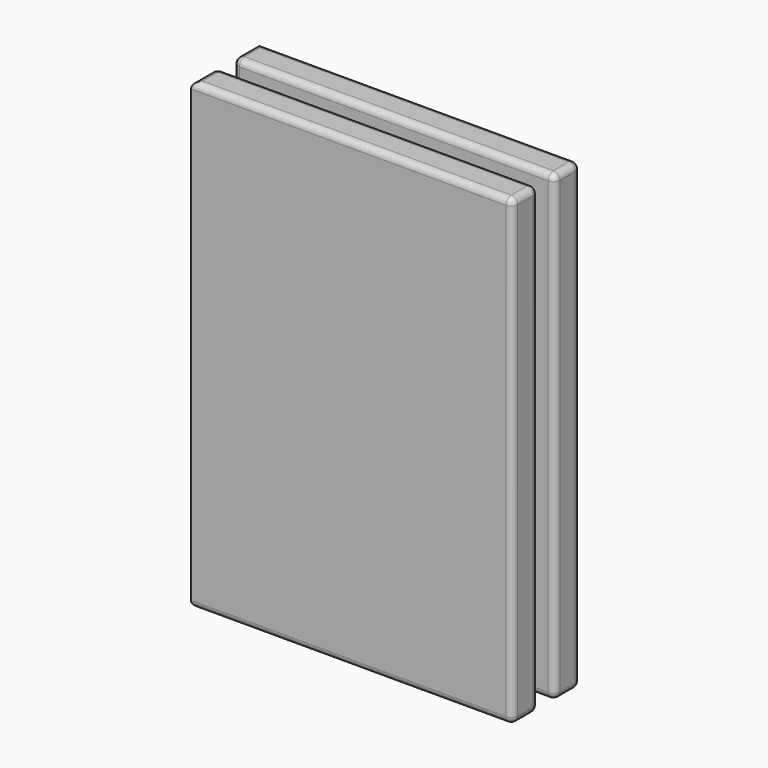
from build123d import *

# Parameters (mm, degrees)
F3_R     = 12.5
F4_DEPTH = 10
F6_DEPTH = 30
F7_R     = 5


with BuildPart() as f2:
    # F2: sweep along a path in F1
    with BuildLine(Plane.XZ) as f2_path:
        Line((0, 0), (250, 0))
    # F0 (on Right) → F2 (sweep)
    with BuildSketch(Plane.YZ):
        Polygon((8, 150), (0, 150), (-8, 150), (-8, 180), (-33, 180), (-33, -180), (-8, -180), (-8, -150), (0, -150), (8, -150), (8, -180), (33, -180), (33, 180), (8, 180), align=None)
    sweep(path=f2_path.line)

    # F3 (on face) → F4 (cut)
    with BuildSketch(Plane(origin=(0, 33, 0), x_dir=(-1, 0, 0), z_dir=(0, 1, 0))):
        with Locations((-60, 150)):
            Circle(F3_R)
        with Locations((-30, 150)):
            Circle(F3_R)
    extrude(amount=-F4_DEPTH, mode=Mode.SUBTRACT)

    # F5 (on face) → F6 (cut)
    with BuildSketch(Plane.YZ.offset(250)):
        Polygon((8, 150), (0, 150), (-8, 150), (-8, -150), (0, -150), (8, -150), align=None)
    extrude(amount=-F6_DEPTH, mode=Mode.SUBTRACT)

    # F7
    f7_edges = [f2.edges().sort_by_distance(p)[0] for p in [
        (110, 8, 150),
        (220, 0, 150),
        (110, -8, 150),
        (0, 0, 150),
        (110, -8, -150),
        (220, 0, -150),
        (110, 8, -150),
        (0, 0, -150),
        (125, 8, -180),
        (0, 20.5, -180),
        (125, 33, -180),
        (250, 20.5, -180),
        (125, 33, 180),
        (0, 20.5, 180),
        (125, 8, 180),
        (250, 20.5, 180),
        (125, -8, 180),
        (0, -20.5, 180),
        (125, -33, 180),
        (250, -20.5, 180),
        (125, -33, -180),
        (0, -20.5, -180),
        (125, -8, -180),
        (250, -20.5, -180),
        (0, -8, 165),
        (0, -8, -165),
        (0, 8, -165),
        (0, 8, 165),
        (250, 8, 0),
        (250, 33, 0),
        (250, -8, 0),
        (250, -33, 0),
        (220, -8, 0),
        (220, 8, 0),
    ]]
    fillet(f7_edges, radius=F7_R)


solid = f2.part
